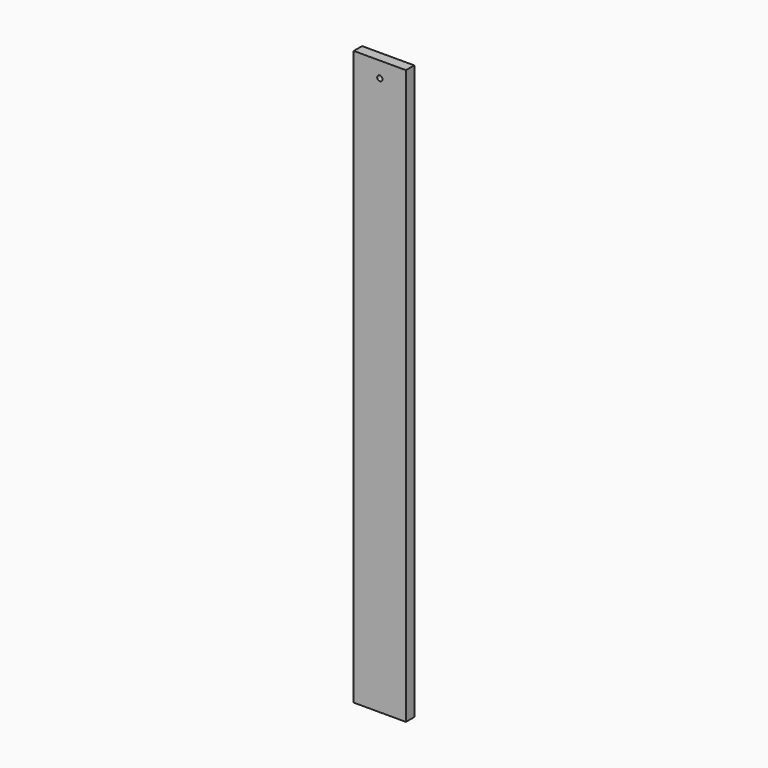
from build123d import *

# Parameters (mm, degrees)
F0_W     = 127
F0_H     = 1397
F0_R     = 6.35
F1_DEPTH = 25.4


# Not quite as in the source:
# - the program builds the solid bodies; features that only make, move or delete a surface that nothing else refers to are left out


with BuildPart() as f1:
    # F0 (on Front) → F1 (new body)
    with BuildSketch(Plane.XZ):
        with Locations((-547.1930051203, 168.3665995002)):
            Rectangle(F0_W, F0_H)
        with Locations((-547.1930051203, 828.7665995002)):
            Circle(F0_R, mode=Mode.SUBTRACT)
    extrude(amount=F1_DEPTH)


solid = f1.part
